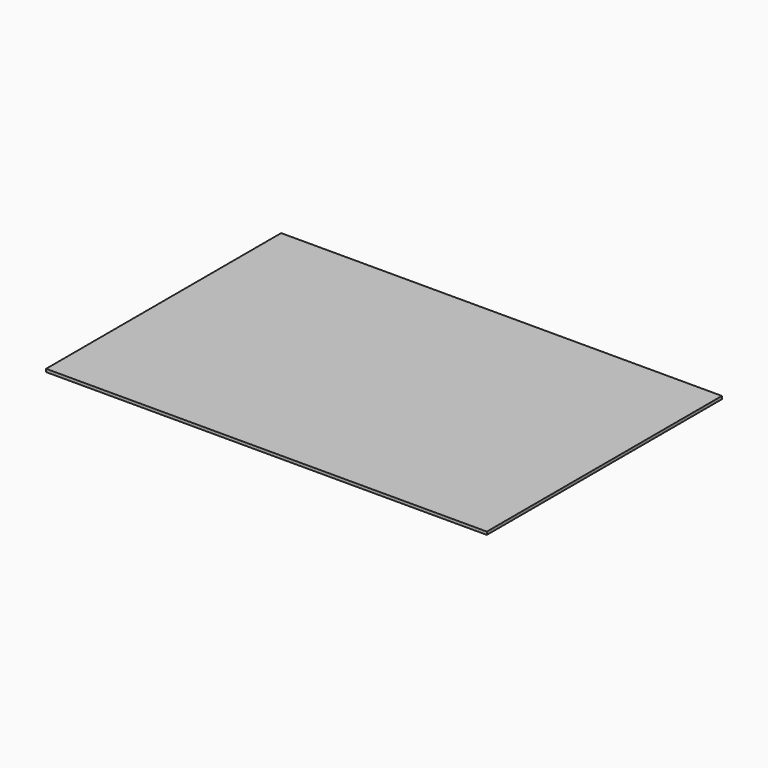
from build123d import *

# Parameters (mm, degrees)
F0_W     = 508
F0_H     = 381
F1_DEPTH = 25.4
F0_W_2   = 254
F0_H_2   = 254
F2_DEPTH = 25.4
F0_W_3   = 381
F0_H_3   = 127
F3_DEPTH = 25.4
F4_DEPTH = 25.4
F0_W_4   = 127
F0_H_4   = 508
F0_W_5   = 635
F5_DEPTH = 25.4
F6_DEPTH = 25.4
F7_DEPTH = 25.4


# Not quite as in the source:
# - a feature names something its author has since deleted; it is built from what else it names


with BuildPart() as f1:
    # F0 (on Top) → F1 (new body)
    with BuildSketch(Plane.XY):
        with Locations((-1016, 1079.5)):
            Rectangle(F0_W, F0_H)
    extrude(amount=F1_DEPTH)

    # F0 (on Top) → F2 (join)
    with BuildSketch(Plane.XY):
        Polygon((-127, 1270), (-762, 1270), (-762, 889), (-762, 508), (-127, 508), (-127, 762), align=None)
        Polygon((127, 1270), (-127, 1270), (-127, 762), (127, 762), (127, 889), align=None)
        Polygon((889, 1270), (127, 1270), (127, 889), (508, 889), (889, 889), align=None)
        Polygon((1397, 1270), (889, 1270), (889, 889), (889, 635), (1270, 635), (1397, 635), (1397, 889), align=None)
        with Locations((1651, 1079.5)):
            Rectangle(F0_W, F0_H)
        Polygon((2540, 1270), (1905, 1270), (1905, 889), (1905, 381), (2286, 381), (2540, 381), align=None)
        Polygon((-762, 889), (-1270, 889), (-1270, 508), (-1016, 508), (-762, 508), align=None)
        Polygon((-127, 508), (-762, 508), (-762, 381), (-127, 381), (508, 381), (508, 508), (127, 508), align=None)
        with Locations((0, 635)):
            Rectangle(F0_W_2, F0_H_2)
        Polygon((127, 889), (127, 762), (127, 508), (508, 508), (508, 889), align=None)
        Polygon((889, 889), (508, 889), (508, 508), (508, 381), (508, 254), (889, 254), (889, 635), align=None)
        Polygon((1270, 635), (889, 635), (889, 254), (889, 127), (1270, 127), align=None)
        Polygon((1397, 635), (1270, 635), (1270, 127), (1270, -127), (1270, -381), (1397, -381), (1397, 0), align=None)
        Polygon((1905, 889), (1397, 889), (1397, 635), (1397, 0), (1651, 0), (1905, 0), (1905, 381), align=None)
        Polygon((2286, 381), (1905, 381), (1905, 0), (1905, -254), (2286, -254), align=None)
        Polygon((2540, -508), (2540, 381), (2286, 381), (2286, -254), (2286, -508), align=None)
    extrude(amount=F2_DEPTH)

    # F0 (on Top) → F3 (join)
    with BuildSketch(Plane.XY):
        Polygon((-1016, 508), (-1270, 508), (-1270, -254), (-1016, -254), (-1016, 254), align=None)
        Polygon((-762, 381), (-762, 508), (-1016, 508), (-1016, 254), (-889, 254), (-762, 254), align=None)
        Polygon((-127, 381), (-762, 381), (-762, 254), (-762, -254), (-127, -254), (-127, 0), align=None)
        Polygon((508, 381), (-127, 381), (-127, 0), (254, 0), (508, 0), (508, 127), (508, 254), align=None)
        with Locations((698.5, 190.5)):
            Rectangle(F0_W_3, F0_H_3)
        Polygon((889, 127), (508, 127), (508, 0), (508, -127), (889, -127), (1270, -127), (1270, 127), align=None)
        with Locations((1079.5, -254)):
            Rectangle(F0_W_3, F0_H_2)
        Polygon((1524, -1016), (1524, -1270), (2032, -1270), (2032, -1016), (1905, -1016), (1651, -1016), align=None)
        Polygon((1651, -381), (1397, -381), (1270, -381), (889, -381), (889, -635), (889, -1016), (1524, -1016), (1651, -1016), (1651, -508), align=None)
        Polygon((1905, -254), (1651, -254), (1651, -381), (1651, -508), (1905, -508), (2286, -508), (2286, -254), align=None)
        Polygon((2540, -1016), (2540, -508), (2286, -508), (1905, -508), (1905, -1016), (2032, -1016), align=None)
    extrude(amount=F3_DEPTH)

    # F0 (on Top) → F4 (join)
    with BuildSketch(Plane.XY):
        Polygon((1651, 0), (1397, 0), (1397, -381), (1651, -381), (1651, -254), align=None)
        with Locations((1778, -127)):
            Rectangle(F0_W_2, F0_H_2)
    extrude(amount=F4_DEPTH)

    # F0 (on Top) → F5 (join)
    with BuildSketch(Plane.XY):
        Polygon((-1016, -254), (-1270, -254), (-1270, -889), (-889, -889), (-889, -254), align=None)
        with Locations((-952.5, 0)):
            Rectangle(F0_W_4, F0_H_4)
        Polygon((-762, -254), (-762, 254), (-889, 254), (-889, -254), (-889, -889), (-762, -889), (-762, -635), align=None)
        Polygon((-127, -254), (-762, -254), (-762, -635), (-254, -635), (-127, -635), (-127, -508), align=None)
        Polygon((254, 0), (-127, 0), (-127, -254), (-127, -508), (254, -508), align=None)
        Polygon((508, 0), (254, 0), (254, -508), (254, -635), (508, -635), (508, -127), align=None)
        Polygon((889, -127), (508, -127), (508, -635), (889, -635), (889, -381), align=None)
        with Locations((1206.5, -1143)):
            Rectangle(F0_W_5, F0_H_2)
        with Locations((1778, -762)):
            Rectangle(F0_W_2, F0_H_4)
        Polygon((1524, -1016), (1524, -1270), (2032, -1270), (2032, -1016), (1905, -1016), (1651, -1016), align=None)
        with Locations((2286, -1143)):
            Rectangle(F0_W, F0_H_2)
    extrude(amount=F5_DEPTH)

    # F0 (on Top) → F6 (join)
    with BuildSketch(Plane.XY):
        Polygon((-889, -889), (-1270, -889), (-1270, -1270), (-762, -1270), (-762, -889), align=None)
        Polygon((-762, -635), (-762, -889), (-762, -1270), (-254, -1270), (-254, -889), (-254, -635), align=None)
        with Locations((-190.5, -762)):
            Rectangle(F0_W_4, F0_H_2)
        Polygon((254, -508), (-127, -508), (-127, -635), (-127, -889), (254, -889), (254, -635), align=None)
        with Locations((381, -762)):
            Rectangle(F0_W_2, F0_H_2)
        Polygon((508, -889), (508, -1270), (889, -1270), (889, -1016), (889, -635), (508, -635), align=None)
    extrude(amount=F6_DEPTH)

    # F0 (on Top) → F7 (join)
    with BuildSketch(Plane.XY):
        Polygon((-254, -889), (-254, -1270), (508, -1270), (508, -889), (254, -889), (-127, -889), align=None)
    extrude(amount=F7_DEPTH)


solid = f1.part
